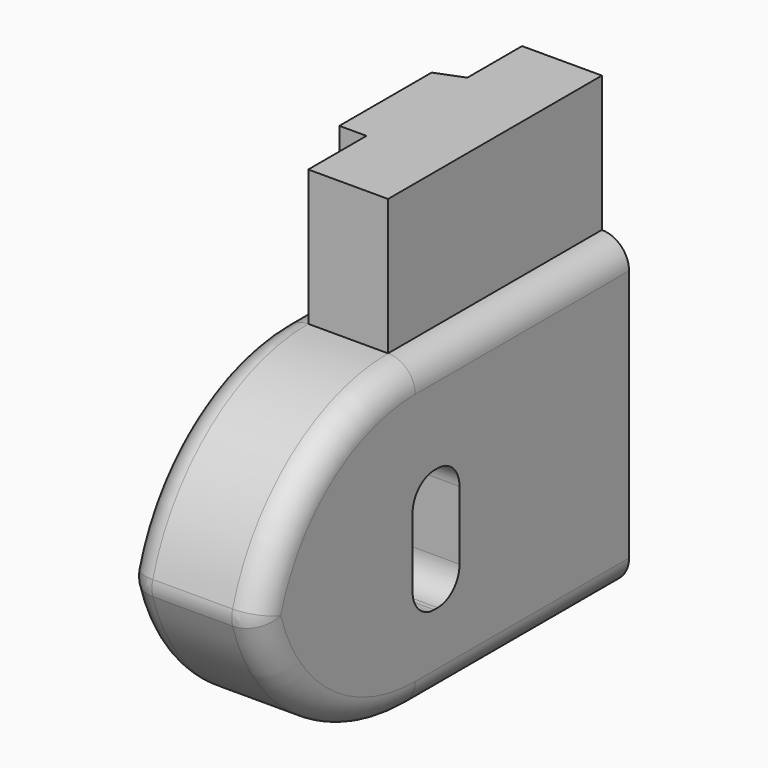
from build123d import *

# Parameters (mm, degrees)
F0_W        = 25.0751823187
F0_H        = 87.748773396
F1_DEPTH    = 57.4051365256
F2_T1_DEPTH = 214.0604270912
F3_R        = 5.08
F4_R        = 5.08
F5_W        = 10.9846293926
F5_H        = 22.9512043297
F6_DEPTH    = 76.7630785704
F7_R        = 5.08
F9_DEPTH    = 36.4525131881
F10_DEPTH   = 25.4


# Not quite as in the source:
# - a fillet or chamfer that OpenCascade refuses, or shapes differently, is made with other operations: its cross-section is extruded or revolved along the edge and cut away or added


with BuildPart() as f1:
    # F0 (on Top) → F1 (new body)
    with BuildSketch(Plane.XY):
        with Locations((12.5375911593, 10.7809714973)):
            Rectangle(F0_W, F0_H)
    extrude(amount=F1_DEPTH)

    # F2: fillet of radius 37.7970489545 on 2 edges, made by hand

    # F2_s2 → F2_t1 (cut)
    with BuildSketch(Plane.YZ.offset(-94.4926223863)):
        with BuildLine():
            ThreePointArc((-33.0934152007, 19.6080875711), (-22.0229158708, 46.3346371957), (4.7036337538, 57.4051365256))
            Line((4.7036337538, 57.4051365256), (-33.0934152007, 57.4051365256))
            Line((-33.0934152007, 57.4051365256), (-33.0934152007, 19.6080875711))
        make_face()
        with BuildLine():
            ThreePointArc((-33.0934152007, 37.7970489545), (-22.0229158708, 11.0704993299), (4.7036337538, 0))
            Line((4.7036337538, 0), (-33.0934152007, 0))
            Line((-33.0934152007, 0), (-33.0934152007, 37.7970489545))
        make_face()
    extrude(amount=F2_T1_DEPTH, mode=Mode.SUBTRACT)

    # F3
    f3_edges = [f1.edges().sort_by_distance(p)[0] for p in [
        (0, 29.679496, 0),
        (0, -18.586626, 8.028261),
        (25.075182, 29.679496, 57.405137),
        (25.075182, -18.586626, 49.376875),
        (25.075182, 29.679496, 0),
        (25.075182, -18.586626, 8.028261),
        (0, -18.586626, 49.376875),
        (0, 29.679496, 57.405137),
    ]]
    fillet(f3_edges, radius=F3_R)

    # F4
    f4_edges = [f1.edges().sort_by_distance(p)[0] for p in [
        (12.537591, -31.982976, 28.702568),
    ]]
    fillet(f4_edges, radius=F4_R)

    # F5 (on face) → F6 (cut)
    with BuildSketch(Plane(origin=(0, 0, 0), x_dir=(0, -1, 0), z_dir=(-1, 0, 0))):
        with Locations((-9.5620453358, 26.5463981777)):
            Rectangle(F5_W, F5_H)
    extrude(amount=-F6_DEPTH, mode=Mode.SUBTRACT)

    # F7
    f7_edges = [f1.edges().sort_by_distance(p)[0] for p in [
        (12.537591, 4.069731, 38.022),
        (12.537591, 4.069731, 15.070796),
        (12.537591, 15.05436, 15.070796),
        (12.537591, 15.05436, 38.022),
    ]]
    fillet(f7_edges, radius=F7_R)

    # F8 (on face) → F9 (join)
    with BuildSketch(Plane.XY.offset(57.4051365256)):
        Polygon((0, 18.3127000928), (5.08, 18.3127000928), (5.08, 41.8710074145), (0, 39.8706048727), align=None)
    extrude(amount=-F9_DEPTH)

    # F10 (add): a face of the model
    f10_faces = [f1.faces().sort_by_distance(p)[0] for p in [
        (11.2098476386, 29.6687845578, 57.4051365256),
    ]]
    extrude(f10_faces, amount=F10_DEPTH)


solid = f1.part
